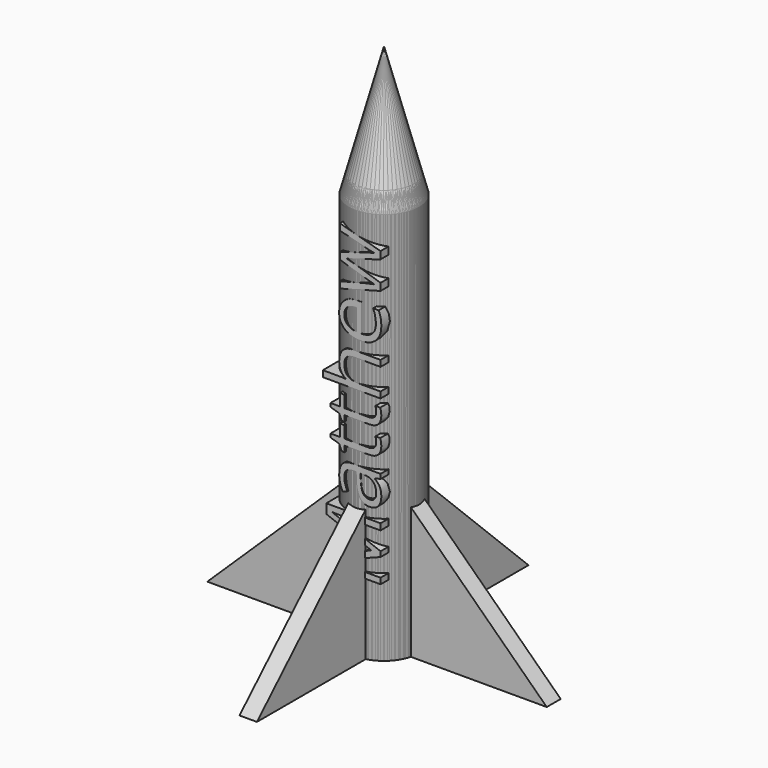
from build123d import *

# Parameters (mm, degrees)
F0_R         = 25.4
F1_DEPTH     = 381
F2_SIZE2     = 94.7940905122
F2_SIZE      = 25.4
F4_DEPTH     = 6.35
F5_COUNT     = 4
F6_TEXT_SIZE = 55.3445373237
F9_DEPTH     = 25.4


# Not quite as in the source:
# - the program builds the solid bodies; features that only make, move or delete a surface that nothing else refers to are left out
# - Text() gives the source's letters only with a copy of the font that has no kerning and outlines rounded to 1/6400 em; it was checked with that copy


with BuildPart() as f1:
    # F0 (on Top) → F1 (new body)
    with BuildSketch(Plane.XY):
        Circle(F0_R)
    extrude(amount=F1_DEPTH)

    # F2
    f2_edges = [f1.edges().sort_by_distance(p)[0] for p in [
        (-25.4, 0, 381),
    ]]
    f2_side = f1.faces().sort_by_distance((0, 0, 381))[0]
    chamfer(f2_edges, length=F2_SIZE, length2=F2_SIZE2, reference=f2_side)

    # F3 (on Front) → F4 (join, symmetric)
    with BuildSketch(Plane.XZ):
        Polygon((0, 119.8220476508), (0, 0), (123.6094459891, 0), align=None)
    extrude(amount=F4_DEPTH, both=True)


with BuildPart() as f5_1:
    # F5: instance of F1
    add(f1.part.rotate(Axis((0, 0, 0), (0, 0, -1)), 1 * 360 / F5_COUNT))


with BuildPart() as f5_2:
    # F5: instance of F1
    add(f1.part.rotate(Axis((0, 0, 0), (0, 0, -1)), 2 * 360 / F5_COUNT))


with BuildPart() as f5_3:
    # F5: instance of F1
    add(f1.part.rotate(Axis((0, 0, 0), (0, 0, -1)), 3 * 360 / F5_COUNT))


with BuildPart() as f9:
    # F6 (on Front) → F9 (new body)
    with BuildSketch(Plane.XZ):
        with Locations(Location((17.8061527194, 46.5871281855), (0, 0, 90))):
            Text('Matthew', F6_TEXT_SIZE, font='Open Sans', text_align=(TextAlign.LEFT, TextAlign.BOTTOM))
    extrude(amount=F9_DEPTH)


solid = Compound([f1.part, f5_1.part, f5_2.part, f5_3.part, f9.part])
